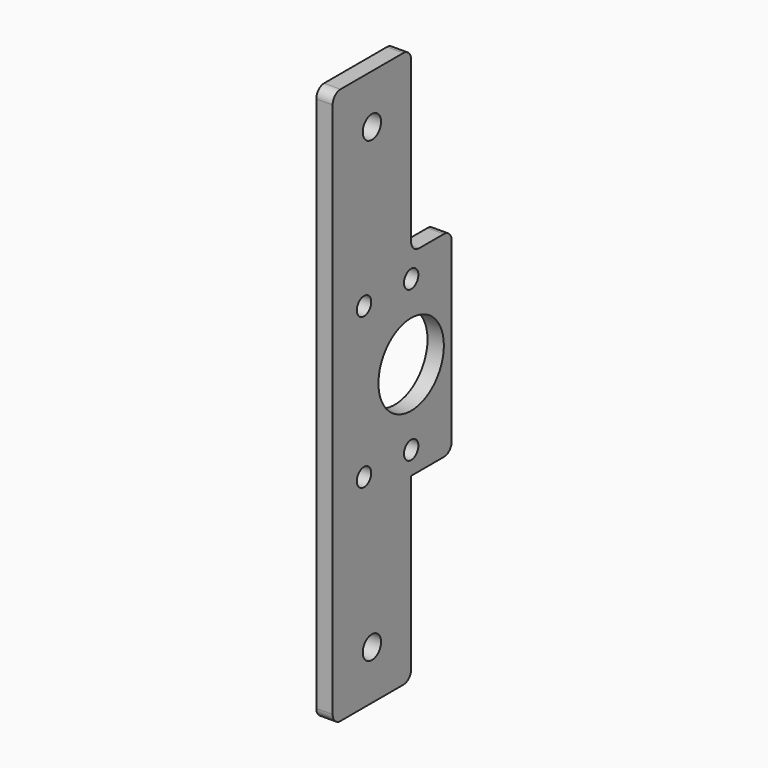
from build123d import *

# Parameters (mm, degrees)
F1_DEPTH = 5
F2_R     = 3
F3_R     = 3.5
F4_DEPTH = 5
F6_R     = 12.5
F6_R_2   = 2.75
F7_DEPTH = 5


# Not quite as in the source:
# - two fillets or chamfers of one size are made in one step


with BuildPart() as f1:
    # F0 (on Right) → F1 (new body)
    with BuildSketch(Plane.YZ):
        Polygon((15, 30), (15, 85), (-15, 85), (-15, -85), (15, -85), (15, -30), (30.5, -30), (30.5, 30), align=None)
    extrude(amount=F1_DEPTH)

    # F2
    f2_edges = [f1.edges().sort_by_distance(p)[0] for p in [
        (2.5, -15, 85),
        (2.5, 15, 85),
        (2.5, -15, -85),
        (2.5, 15, 30),
        (2.5, 15, -85),
        (2.5, 30.5, -30),
        (2.5, 30.5, 30),
    ]]
    fillet(f2_edges, radius=F2_R)

    # F3 (on face) → F4 (cut)
    with BuildSketch(Plane.YZ.offset(5)):
        with Locations((0, 70)):
            Circle(F3_R)
        with Locations((0, -70)):
            Circle(F3_R)
    extrude(amount=-F4_DEPTH, mode=Mode.SUBTRACT)

    # F6 (on face) → F7 (cut)
    with BuildSketch(Plane.YZ.offset(5)):
        with Locations((15, 0)):
            Circle(F6_R)
        with Locations((15, 23)):
            Circle(F6_R_2)
        with Locations((15, -23)):
            Circle(F6_R_2)
        with Locations((-3, -23)):
            Circle(F6_R_2)
        with Locations((-3, 23)):
            Circle(F6_R_2)
    extrude(amount=-F7_DEPTH, mode=Mode.SUBTRACT)


solid = f1.part
